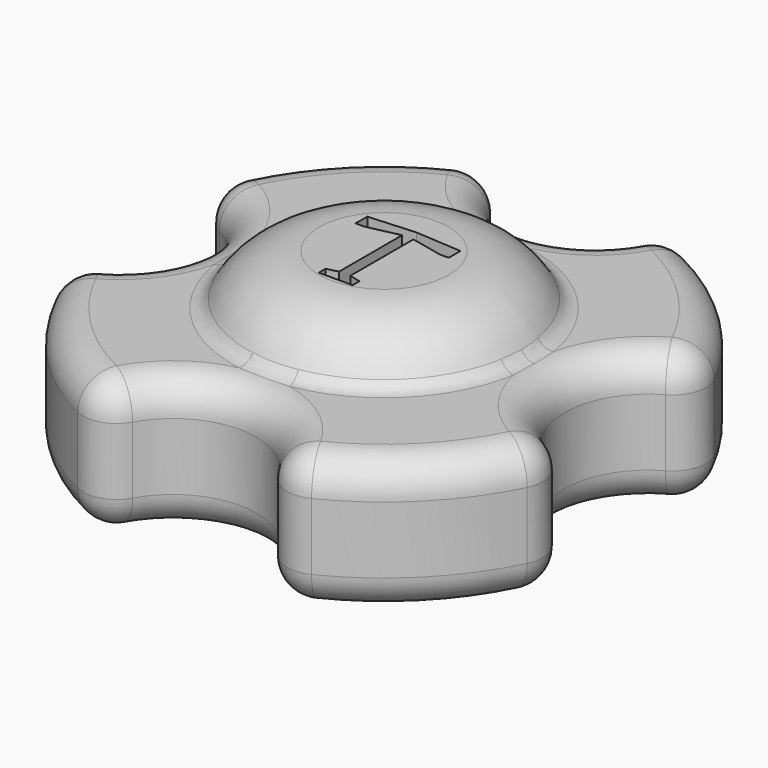
from build123d import *

# Parameters (mm, degrees)
F1_DEPTH = 8
F2_R     = 2
F3_R     = 2
F4_R     = 8.4594661891
F5_DEPTH = 3
F7_R     = 1
F9_DEPTH = 1


# Not quite as in the source:
# - a fillet or chamfer that OpenCascade refuses, or shapes differently, is made with other operations: its cross-section is extruded or revolved along the edge and cut away or added


with BuildPart() as f1:
    # F0 (on Top) → F1 (new body)
    with BuildSketch(Plane.XY):
        with BuildLine():
            ThreePointArc((-4.3603955862, 13.336509077), (-5.5129295549, 14.2682715346), (-6.9903415394, 14.1509273633))
            ThreePointArc((-6.9903415394, 14.1509273633), (-11.1605022306, 11.1605022306), (-14.1509273633, 6.9903415394))
            ThreePointArc((-14.1509273633, 6.9903415394), (-14.2682715346, 5.5129295549), (-13.336509077, 4.3603955862))
            ThreePointArc((-13.336509077, 4.3603955862), (-10.7833336174, 0), (-13.336509077, -4.3603955862))
            ThreePointArc((-13.336509077, -4.3603955862), (-14.2682715346, -5.5129295549), (-14.1509273633, -6.9903415394))
            ThreePointArc((-14.1509273633, -6.9903415394), (-11.1605022306, -11.1605022306), (-6.9903415394, -14.1509273633))
            ThreePointArc((-6.9903415394, -14.1509273633), (-5.5129295549, -14.2682715346), (-4.3603955862, -13.336509077))
            ThreePointArc((-4.3603955862, -13.336509077), (0, -10.7833336174), (4.3603955862, -13.336509077))
            ThreePointArc((4.3603955862, -13.336509077), (5.5129295549, -14.2682715346), (6.9903415394, -14.1509273633))
            ThreePointArc((6.9903415394, -14.1509273633), (11.1605022306, -11.1605022306), (14.1509273633, -6.9903415394))
            ThreePointArc((14.1509273633, -6.9903415394), (14.2682715346, -5.5129295549), (13.336509077, -4.3603955862))
            ThreePointArc((13.336509077, -4.3603955862), (10.7833336174, 0), (13.336509077, 4.3603955862))
            ThreePointArc((13.336509077, 4.3603955862), (14.2682715346, 5.5129295549), (14.1509273633, 6.9903415394))
            ThreePointArc((14.1509273633, 6.9903415394), (11.1605022306, 11.1605022306), (6.9903415394, 14.1509273633))
            ThreePointArc((6.9903415394, 14.1509273633), (5.5129295549, 14.2682715346), (4.3603955862, 13.336509077))
            ThreePointArc((4.3603955862, 13.336509077), (0, 10.7833336174), (-4.3603955862, 13.336509077))
        make_face()
        Polygon((-5.8312377188, 0), (-2.9156188594, 5.05), (2.9156188594, 5.05), (5.8312377188, 0), (2.9156188594, -5.05), (-2.9156188594, -5.05), align=None, mode=Mode.SUBTRACT)
    extrude(amount=F1_DEPTH)

    # F2
    f2_edges = [f1.edges().sort_by_distance(p)[0] for p in [
        (11.160502, 11.160502, 8),
        (0, 10.783334, 8),
        (5.51293, 14.268272, 8),
        (-5.51293, 14.268272, 8),
        (-11.160502, 11.160502, 8),
        (-14.268272, 5.51293, 8),
        (-10.783334, 0, 8),
        (14.268272, 5.51293, 8),
        (10.783334, 0, 8),
        (14.268272, -5.51293, 8),
        (11.160502, -11.160502, 8),
        (-14.268272, -5.51293, 8),
        (-11.160502, -11.160502, 8),
        (0, -10.783334, 8),
        (-5.51293, -14.268272, 8),
        (5.51293, -14.268272, 8),
    ]]
    fillet(f2_edges, radius=F2_R)

    # F3
    f3_edges = [f1.edges().sort_by_distance(p)[0] for p in [
        (11.160502, 11.160502, 0),
        (14.268272, 5.51293, 0),
        (10.783334, 0, 0),
        (14.268272, -5.51293, 0),
        (11.160502, -11.160502, 0),
        (5.51293, -14.268272, 0),
        (0, -10.783334, 0),
        (-5.51293, -14.268272, 0),
        (-11.160502, -11.160502, 0),
        (-14.268272, -5.51293, 0),
        (-10.783334, 0, 0),
        (-14.268272, 5.51293, 0),
        (-11.160502, 11.160502, 0),
        (-5.51293, 14.268272, 0),
        (0, 10.783334, 0),
        (5.51293, 14.268272, 0),
    ]]
    fillet(f3_edges, radius=F3_R)

    # F4 (on face) → F5 (join)
    with BuildSketch(Plane.XY.offset(8)):
        Circle(F4_R)
    extrude(amount=F5_DEPTH)

    # F6: fillet of radius 5 on 1 edges, made by hand

    # F6_s1 → F6_t2 (revolve, cut)
    with BuildSketch(Plane.XZ):
        with BuildLine():
            ThreePointArc((8.4594661891, 8), (6.6155032816, 10.1833001327), (3.8768904941, 11))
            Line((3.8768904941, 11), (8.4594661891, 11))
            Line((8.4594661891, 11), (8.4594661891, 8))
        make_face()
    revolve(axis=Axis((0, 0, 11), (0, 0, 1)), mode=Mode.SUBTRACT)

    # F7
    f7_edges = [f1.edges().sort_by_distance(p)[0] for p in [
        (-8.459466, 0, 8),
    ]]
    fillet(f7_edges, radius=F7_R)

    # F8 (on face) → F9 (cut)
    with BuildSketch(Plane.XY.offset(11)):
        Polygon((-1.0127555579, -3.6138410214), (0, -3.6138410214), (1.0127555579, -3.6138410214), (1.0127555579, -3.1025193166), (0.3370805643, -2.9381657951), (0.3370805643, 1.7732984852), (2.2727984469, 1.3532845769), (2.7841201518, 1.3532845769), (2.7841201518, 2.2298358381), (0, 2.4124509655), (-2.7841201518, 2.2298358381), (-2.7841201518, 1.3532845769), (-2.2727984469, 1.3532845769), (-0.3370805643, 1.7732984852), (-0.3370805643, -2.9381657951), (-1.0127555579, -3.1025193166), align=None)
    extrude(amount=-F9_DEPTH, mode=Mode.SUBTRACT)


solid = f1.part
